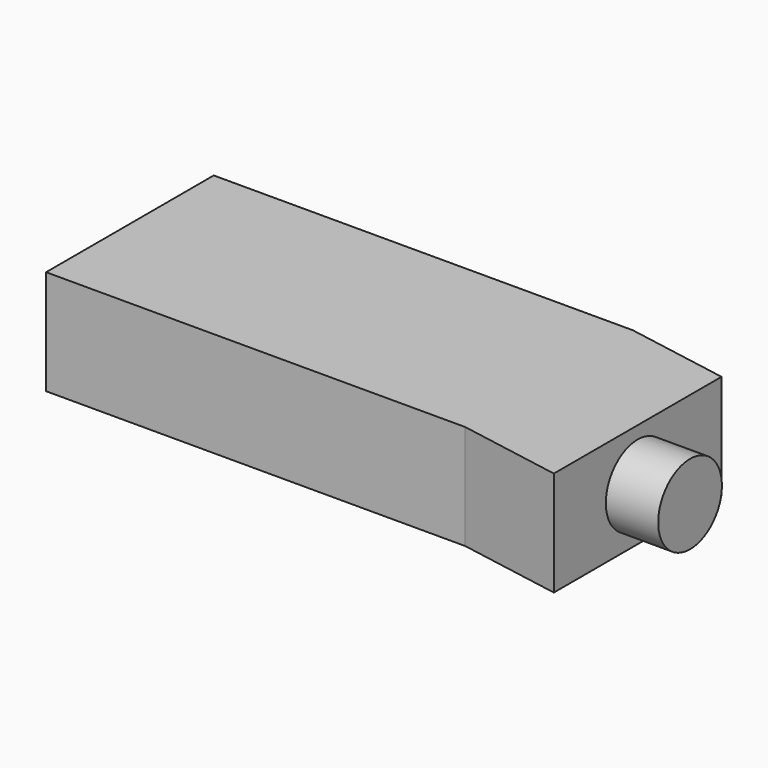
from build123d import *

# Parameters (mm, degrees)
F0_W     = 50.8
F0_H     = 25.4
F1_DEPTH = 12.7
F2_R     = 4.826
F3_DEPTH = 6.35


# Not quite as in the source:
# - a feature names something its author has since deleted; it is built from what else it names


with BuildPart() as f1:
    # F0 (on Top) → F1 (new body)
    with BuildSketch(Plane.XY):
        Rectangle(F0_W, F0_H)
        Polygon((37.9070584633, 10.4946681436), (25.4, 12.7), (25.4, -12.7), (37.9070584633, -14.9053318564), (37.9070584633, -2.2053318564), align=None)
    extrude(amount=-F1_DEPTH)

    # F2 (on face) → F3 (join)
    with BuildSketch(Plane.YZ.offset(37.9070584633)):
        with Locations((-2.2053318564, -6.35)):
            Circle(F2_R)
    extrude(amount=F3_DEPTH)


solid = f1.part
